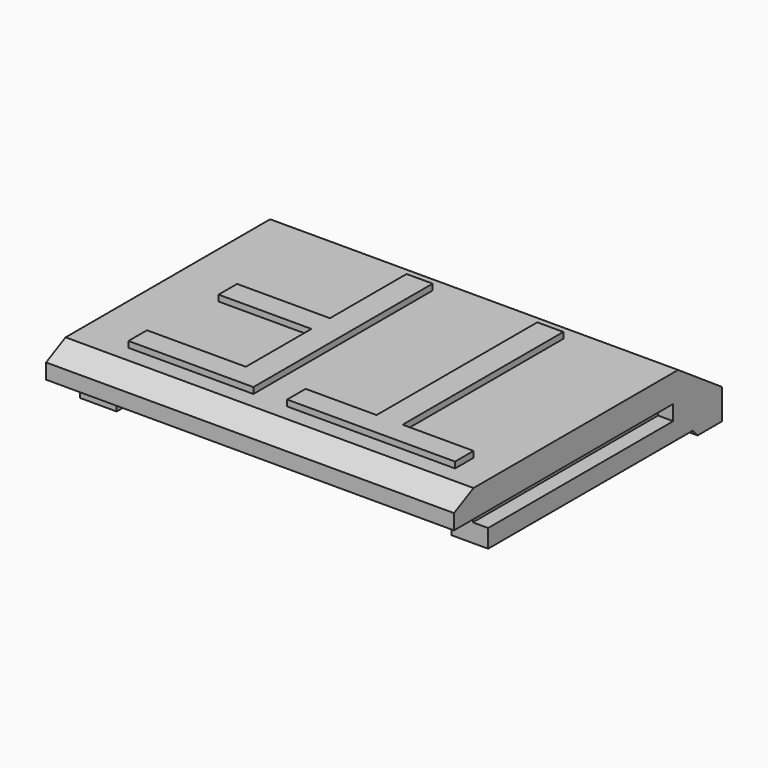
from build123d import *

# Parameters (mm, degrees)
F0_W          = 17.018
F0_H          = 13.97
F1_DEPTH      = 2.54
F3_DEPTH      = 17.018
F5_DEPTH      = 17.018
F6_W          = 0.635
F6_H          = 0.635
F7_DEPTH      = 11.43
F8_W          = 1.778
F8_H          = 0.635
F8_H_2        = 0.762
F9_DEPTH      = 17.018
F10_W         = 13.97
F10_H         = 10.668
F11_DEPTH     = 1.397
F13_DEPTH     = 17.018
F14_TEXT_SIZE = 13.0916788605
F15_DEPTH     = 0.254


# Not quite as in the source:
# - Text() gives the source's letters only with a copy of the font that has no kerning and outlines rounded to 1/6400 em; it was checked with that copy


with BuildPart() as f1:
    # F0 (on Top) → F1 (new body)
    with BuildSketch(Plane.XY):
        Rectangle(F0_W, F0_H)
    extrude(amount=F1_DEPTH)

    # F2 (on face) → F3 (join, through all)
    with BuildSketch(Plane.YZ.offset(8.509)):
        Polygon((6.985, -0.2794), (6.985, 0), (5.461, 0), (5.715, -0.2794), align=None)
    extrude(amount=-F3_DEPTH)

    # F4 (on face) → F5 (cut, through all)
    with BuildSketch(Plane.YZ.offset(8.509)):
        Polygon((6.985, 2.54), (4.699, 2.54), (6.985, 0.9906), align=None)
    extrude(amount=-F5_DEPTH, mode=Mode.SUBTRACT)

    # F6 (on face) → F7 (cut)
    with BuildSketch(Plane.XZ.offset(6.985)):
        with Locations((-8.1915, 1.0795)):
            Rectangle(F6_W, F6_H)
        with Locations((8.1915, 1.0795)):
            Rectangle(F6_W, F6_H)
    extrude(amount=-F7_DEPTH, mode=Mode.SUBTRACT)

    # F8 (on face) → F9 (cut, through all)
    with BuildSketch(Plane.YZ.offset(8.509)):
        with Locations((-6.096, 1.0795)):
            Rectangle(F8_W, F8_H)
        with Locations((-6.096, 0.381)):
            Rectangle(F8_W, F8_H_2)
    extrude(amount=-F9_DEPTH, mode=Mode.SUBTRACT)

    # F10 (on face) → F11 (cut, through all)
    with BuildSketch(Plane(origin=(0, 0, 0), x_dir=(1, 0, 0), z_dir=(0, 0, -1))):
        with Locations((0, -0.127)):
            Rectangle(F10_W, F10_H)
    extrude(amount=-F11_DEPTH, mode=Mode.SUBTRACT)

    # F12 (on face) → F13 (cut, through all)
    with BuildSketch(Plane.YZ.offset(8.509)):
        Polygon((-6.985, 2.54), (-6.985, 2.032), (-5.969, 2.54), align=None)
    extrude(amount=-F13_DEPTH, mode=Mode.SUBTRACT)

    # F14 (on face) → F15 (join)
    with BuildSketch(Plane.XY.offset(2.54)):
        with Locations(Location((7.2934970277, 4.0780043898), (0, 0, -180))):
            Text('TF', F14_TEXT_SIZE, font='Open Sans', text_align=(TextAlign.LEFT, TextAlign.BOTTOM))
    extrude(amount=F15_DEPTH)


solid = f1.part
